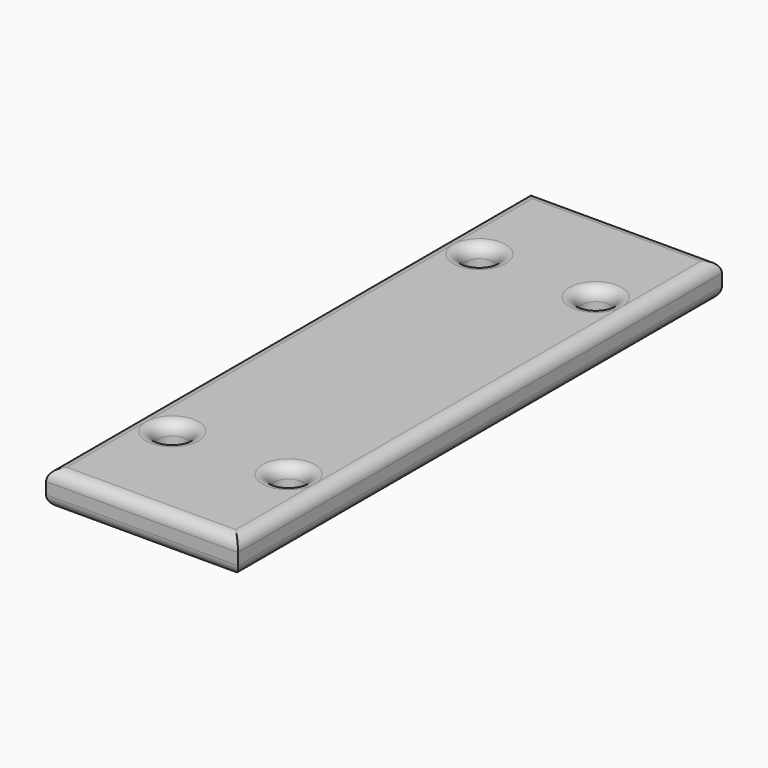
from build123d import *

# Parameters (mm, degrees)
F0_W     = 16.5
F0_H     = 52
F0_R     = 1.25
F1_DEPTH = 3
F2_R     = 0.99999


# Not quite as in the source:
# - a fillet or chamfer is up to 0.001 mm smaller than in the source, because OpenCascade refuses the exact size


with BuildPart() as f1:
    # F0 (on Top) → F1 (new body)
    with BuildSketch(Plane.XY):
        with Locations((8.25, 26)):
            Rectangle(F0_W, F0_H)
        with Locations((3.25, 9.5)):
            Circle(F0_R, mode=Mode.SUBTRACT)
        with Locations((13.25, 9.5)):
            Circle(F0_R, mode=Mode.SUBTRACT)
        with Locations((3.25, 42.5)):
            Circle(F0_R, mode=Mode.SUBTRACT)
        with Locations((13.25, 42.5)):
            Circle(F0_R, mode=Mode.SUBTRACT)
    extrude(amount=F1_DEPTH)

    # F2 (radius 1 in the source; OpenCascade refuses exactly that, so slightly less here)
    f2_edges = [f1.edges().sort_by_distance(p)[0] for p in [
        (16.5, 26, 3),
        (8.25, 52, 3),
        (0, 26, 3),
        (8.25, 0, 3),
        (2, 9.5, 3),
        (12, 9.5, 3),
        (2, 42.5, 3),
        (12, 42.5, 3),
        (16.5, 26, 0),
        (8.25, 52, 0),
        (0, 26, 0),
        (8.25, 0, 0),
    ]]
    fillet(f2_edges, radius=F2_R)


solid = f1.part
